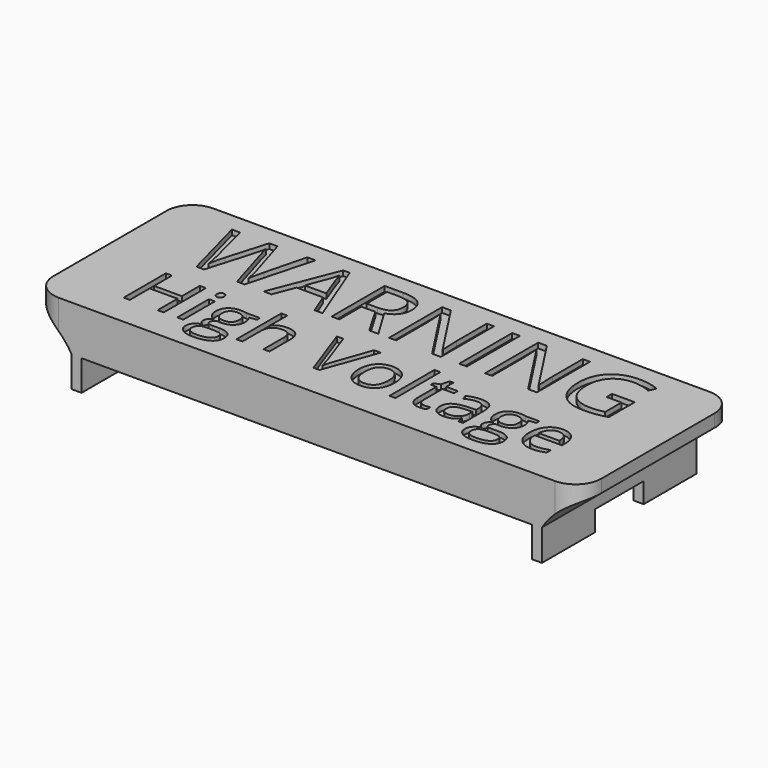
from build123d import *

# Parameters (mm, degrees)
F0_W           = 92.5
F0_H           = 38
F0_W_2         = 88.5
F0_H_2         = 34
F1_DEPTH       = 12
F2_W           = 88.5
F2_H           = 12
F3_DEPTH       = 48.26
F4_W           = 92.5
F4_H           = 38
F5_DEPTH       = 3
F6_TEXT_SIZE   = 18.2736522725
F6_TEXT_SIZE_2 = 14.5169144713
F7_DEPTH       = 1
F9_DEPTH       = 19
F9_DEPTH_BACK  = 19
F10_R          = 5.08
F11_W          = 12
F11_H          = 4
F12_DEPTH      = 100.1210001


# Not quite as in the source:
# - Text() gives the source's letters only with a copy of the font that has no kerning and outlines rounded to 1/6400 em; it was checked with that copy


with BuildPart() as f1:
    # F0 (on Top) → F1 (new body)
    with BuildSketch(Plane.XY):
        Rectangle(F0_W, F0_H)
        Rectangle(F0_W_2, F0_H_2, mode=Mode.SUBTRACT)
    extrude(amount=F1_DEPTH)

    # F2 (on face) → F3 (cut)
    with BuildSketch(Plane.XZ.offset(19)):
        Rectangle(F2_W, F2_H)
    extrude(amount=-F3_DEPTH, mode=Mode.SUBTRACT)

    # F4 (on face) → F5 (join)
    with BuildSketch(Plane.XY.offset(12)):
        Rectangle(F4_W, F4_H)
    extrude(amount=F5_DEPTH)

    # F6 (on face) → F7 (cut)
    with BuildSketch(Plane.XY.offset(15)):
        with Locations((-42.403947562, 2.2869703638)):
            Text('WARNING', F6_TEXT_SIZE, font='Open Sans', text_align=(TextAlign.LEFT, TextAlign.BOTTOM))
        with Locations((-42.403947562, -12.7372080556)):
            Text('High Voltage', F6_TEXT_SIZE_2, font='Open Sans', text_align=(TextAlign.LEFT, TextAlign.BOTTOM))
    extrude(amount=-F7_DEPTH, mode=Mode.SUBTRACT)

    # F8 (on Front) → F9 (join, two sides)
    with BuildSketch(Plane.XZ) as f9_sk:
        with BuildLine():
            Line((-46.25, 6.1412781328), (-46.25, 15))
            Line((-46.25, 15), (-53.87, 15))
            Line((-53.87, 15), (-53.87, 12.496717602))
            ThreePointArc((-53.87, 12.496717602), (-49.5555343573, 9.9238385265), (-46.25, 6.1412781328))
        make_face()
        with BuildLine():
            Line((46.25, 15), (46.25, 6.1412781328))
            ThreePointArc((46.25, 6.1412781328), (49.5555343573, 9.9238385265), (53.87, 12.496717602))
            Line((53.87, 12.496717602), (53.87, 15))
            Line((53.87, 15), (46.25, 15))
        make_face()
    extrude(amount=F9_DEPTH)
    extrude(f9_sk.sketch, amount=-F9_DEPTH_BACK)

    # F10
    f10_edges = [f1.edges().sort_by_distance(p)[0] for p in [
        (-53.87, -19, 13.748359),
        (-53.87, 19, 13.748359),
        (53.87, -19, 13.748359),
        (53.87, 19, 13.748359),
    ]]
    fillet(f10_edges, radius=F10_R)

    # F11 (on face) → F12 (cut, through all)
    with BuildSketch(Plane(origin=(-46.25, 0, 0), x_dir=(0, -1, 0), z_dir=(-1, 0, 0))):
        with Locations((0, 2)):
            Rectangle(F11_W, F11_H)
    extrude(amount=-F12_DEPTH, mode=Mode.SUBTRACT)


solid = f1.part
